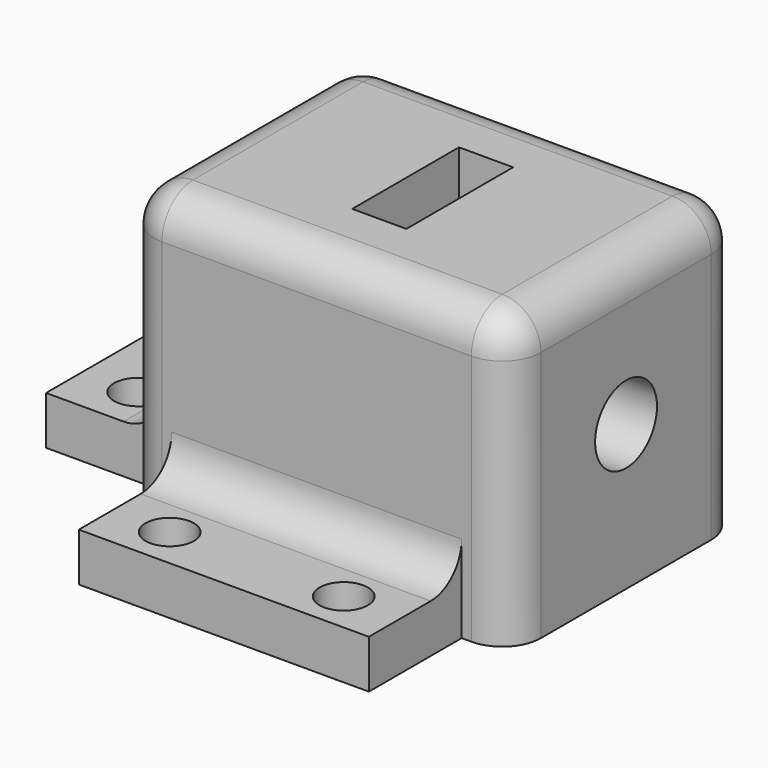
from build123d import *

# Parameters (mm, degrees)
F1_DEPTH = 30
F0_W     = 30
F0_H     = 12
F2_DEPTH = 5
F3_R     = 4
F4_DEPTH = 40.001
F5_R     = 2.5
F6_DEPTH = 5.001
F7_W     = 5.6
F7_H     = 13.8
F8_DEPTH = 30.001
F0_W_2   = 12
F0_H_2   = 20
F0_R     = 2.5
F9_DEPTH = 5
F10_R    = 4


# Not quite as in the source:
# - a feature names something its author has since deleted; it is built from what else it names


with BuildPart() as f1:
    # F0 (on Top) → F1 (new body)
    with BuildSketch(Plane.XY):
        Polygon((15, -15), (20, -15), (20, 15), (-20, 15), (-20, 10.0191985071), (-20, -9.9808014929), (-20, -15), (-15, -15), align=None)
    extrude(amount=F1_DEPTH)

    # F0 (on Top) → F2 (join)
    with BuildSketch(Plane.XY):
        with Locations((0, -21)):
            Rectangle(F0_W, F0_H)
    extrude(amount=F2_DEPTH)

    # F3 (on face) → F4 (cut, through all)
    with BuildSketch(Plane.YZ.offset(20)):
        with Locations((0, 15)):
            Circle(F3_R)
    extrude(amount=-F4_DEPTH, mode=Mode.SUBTRACT)

    # F5 (on face) → F6 (cut, through all)
    with BuildSketch(Plane.XY.offset(5)):
        with Locations((9, -22.75)):
            Circle(F5_R)
        with Locations((-9, -22.75)):
            Circle(F5_R)
    extrude(amount=-F6_DEPTH, mode=Mode.SUBTRACT)

    # F7 (on face) → F8 (cut, through all)
    with BuildSketch(Plane.XY.offset(30)):
        Rectangle(F7_W, F7_H)
    extrude(amount=-F8_DEPTH, mode=Mode.SUBTRACT)

    # F0 (on Top) → F9 (join)
    with BuildSketch(Plane.XY):
        with Locations((-26, 0.0191985071)):
            Rectangle(F0_W_2, F0_H_2)
        with Locations((-26.2869596481, -5.2162762731)):
            Circle(F0_R, mode=Mode.SUBTRACT)
        with Locations((-26.2869596481, 5.0912299193)):
            Circle(F0_R, mode=Mode.SUBTRACT)
    extrude(amount=F9_DEPTH)

    # F10
    f10_edges = [f1.edges().sort_by_distance(p)[0] for p in [
        (-20, 0.019199, 5),
        (-20, 15, 15),
        (-20, 0, 30),
        (-20, -15, 15),
        (0, -15, 5),
        (0, -15, 30),
        (20, -15, 15),
        (20, 0, 30),
        (0, 15, 30),
        (20, 15, 15),
    ]]
    fillet(f10_edges, radius=F10_R)


solid = f1.part
